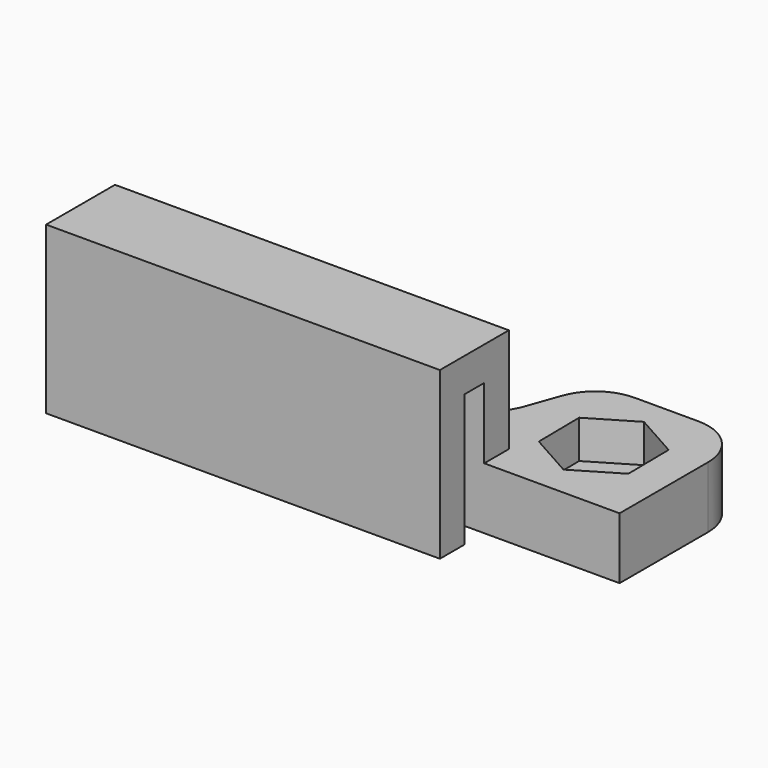
from build123d import *

# Parameters (mm, degrees)
F1_DEPTH  = 5
F3_DEPTH  = 3.1
F4_R      = 2.25
F5_DEPTH  = 5.001
F6_W      = 32
F6_H      = 2.5
F7_DEPTH  = 8.5
F8_W      = 32
F8_H      = 2.75
F9_DEPTH  = 4.5
F10_W     = 32
F10_H     = 2.5
F11_DEPTH = 10.75
F12_R     = 1.35
F13_DEPTH = 3
F14_DEPTH = 2.5


# Not quite as in the source:
# - a feature names something its author has since deleted; it is built from what else it names


with BuildPart() as f1:
    # F0 (on Top) → F1 (new body)
    with BuildSketch(Plane.XY):
        with BuildLine():
            Line((0, 2.5), (0, 0))
            Line((0, 0), (43, 0))
            Line((43, 0), (43, 9))
            ThreePointArc((43, 9), (41.8284271247, 11.8284271247), (39, 13))
            Line((39, 13), (33.8239016482, 13))
            ThreePointArc((33.8239016482, 13), (31.5169659003, 12.2677281794), (30.0546821723, 10.3390237274))
            Line((30.0546821723, 10.3390237274), (29.1077482568, 7.6734983272))
            ThreePointArc((29.1077482568, 7.6734983272), (27.8028764103, 5.8618093159), (25.7302204856, 5.0317460488))
            Line((25.7302204856, 5.0317460488), (0, 2.5))
        make_face()
    extrude(amount=F1_DEPTH)

    # F2 (on face) → F3 (cut)
    with BuildSketch(Plane.XY.offset(5)):
        Polygon((39.9846022951, 8.7502746915), (36.3578632635, 10.7817185123), (32.7852117926, 8.6565922885), (32.8392993532, 4.5000222439), (36.4660383847, 2.4685784231), (40.0386898557, 4.5937046469), align=None)
    extrude(amount=-F3_DEPTH, mode=Mode.SUBTRACT)

    # F4 (on face) → F5 (cut, through all)
    with BuildSketch(Plane(origin=(0, 0, 0), x_dir=(1, 0, 0), z_dir=(0, 0, -1))):
        with Locations((36.4119508241, -6.4989285606)):
            Circle(F4_R)
    extrude(amount=-F5_DEPTH, mode=Mode.SUBTRACT)

    # F6 (on face) → F7 (join)
    with BuildSketch(Plane.XY.offset(5)):
        with Locations((16, 1.25)):
            Rectangle(F6_W, F6_H)
    extrude(amount=F7_DEPTH)

    # F8 (on face) → F9 (join)
    with BuildSketch(Plane.XZ):
        with Locations((16, 12.125)):
            Rectangle(F8_W, F8_H)
    extrude(amount=F9_DEPTH)

    # F10 (on face) → F11 (join)
    with BuildSketch(Plane(origin=(0, 0, 10.75), x_dir=(1, 0, 0), z_dir=(0, 0, -1))):
        with Locations((16, 3.25)):
            Rectangle(F10_W, F10_H)
    extrude(amount=F11_DEPTH)

    # F12 (on face) → F13 (join)
    with BuildSketch(Plane(origin=(0, 2.5, 0), x_dir=(-1, 0, 0), z_dir=(0, 1, 0))):
        with BuildLine():
            Line((-27.1456439237, 5), (-24.8543560763, 5))
            ThreePointArc((-24.8543560763, 5), (-26, 10.25), (-27.1456439237, 5))
        make_face()
        with Locations((-26, 7.5)):
            Circle(F12_R, mode=Mode.SUBTRACT)
        with BuildLine():
            Line((-7.1456439237, 5), (-4.8543560763, 5))
            ThreePointArc((-4.8543560763, 5), (-6, 10.25), (-7.1456439237, 5))
        make_face()
        with Locations((-6, 7.5)):
            Circle(F12_R, mode=Mode.SUBTRACT)
    extrude(amount=F13_DEPTH)

    # F14 (cut, through all): faces of the model
    f14_faces = [f1.faces().sort_by_distance(p)[0] for p in [
        (6, 2.5, 7.5),
        (26, 2.5, 7.5),
    ]]
    extrude(f14_faces, amount=-F14_DEPTH, mode=Mode.SUBTRACT)


solid = f1.part
